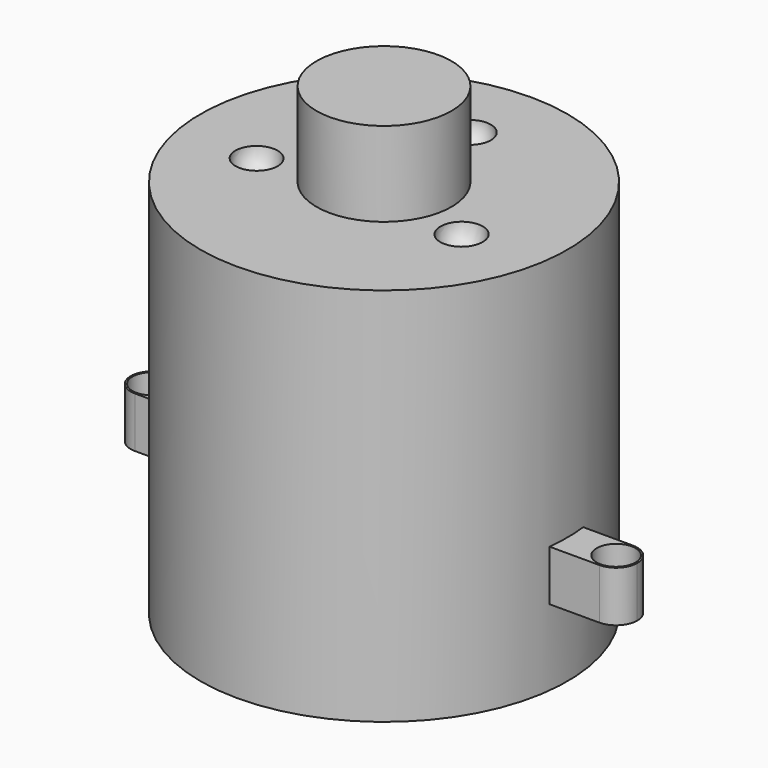
from build123d import *

# Parameters (mm, degrees)
F0_W     = 8
F0_H     = 10
F2_W     = 60
F2_H     = 6
F3_DEPTH = 2.5
F4_R     = 2.49999
F6_D     = 4.6
F6_DEPTH = 4
F6_TIP   = 1.3819794238


# Not quite as in the source:
# - a fillet or chamfer is up to 0.001 mm smaller than in the source, because OpenCascade refuses the exact size


with BuildPart() as f1:
    # F0 (on Right) → F1 (revolve)
    with BuildSketch(Plane.YZ):
        Polygon((-21.75, 22.5), (-21.75, -22.5), (0, -22.5), (0, 22.5), (-8, 22.5), align=None)
        with Locations((-4, 27.5)):
            Rectangle(F0_W, F0_H)
    revolve(axis=Axis((0, 0, 5), (0, 0, -1)))

    # F2 (on Front) → F3 (join, symmetric)
    with BuildSketch(Plane.XZ):
        with Locations((0, -10.5)):
            Rectangle(F2_W, F2_H)
    extrude(amount=F3_DEPTH, both=True)

    # F4 (radius 2.5 in the source; OpenCascade refuses exactly that, so slightly less here)
    f4_edges = [f1.edges().sort_by_distance(p)[0] for p in [
        (30, 2.5, -10.5),
        (-30, 2.5, -10.5),
        (30, -2.5, -10.5),
        (-30, -2.5, -10.5),
    ]]
    fillet(f4_edges, radius=F4_R)

    # F6
    with Locations(Plane.XY.offset(-7.5)):
        with Locations((-27.5, 0), (27.5, 0)):
            Hole(F6_D / 2, depth=F6_DEPTH)
            with Locations((0, 0, -(F6_DEPTH + F6_TIP / 2))):  # 118° drill point
                Cone(0, F6_D / 2, F6_TIP, mode=Mode.SUBTRACT)

    # F7 (on face) → F8 (revolve, cut)
    with BuildSketch(Plane.XY.offset(22.5)):
        with BuildLine():
            ThreePointArc((0, 10.197782052), (1.767766953, 10.9300150991), (2.5, 12.697782052))
            ThreePointArc((2.5, 12.697782052), (1.767766953, 14.465549005), (0, 15.197782052))
            Line((0, 15.197782052), (0, 10.197782052))
        make_face()
    revolve(axis=Axis((0, 12.697782052, 22.5), (0, -1, 0)), mode=Mode.SUBTRACT)

    # F7 (on face) → F9 (revolve, cut)
    with BuildSketch(Plane.XY.offset(22.5)):
        with BuildLine():
            Line((-14.6499237033, -3.669800331), (-9.65, -3.6893317878))
            ThreePointArc((-9.65, -3.6893317878), (-12.1402341971, -1.1893508621), (-14.6499237033, -3.669800331))
        make_face()
    revolve(axis=Axis((-12.1499618516, -3.6795660594, 22.5), (0.9999923703, -0.0039063212, 0)), mode=Mode.SUBTRACT)

    # F7 (on face) → F10 (revolve, cut)
    with BuildSketch(Plane.XY.offset(22.5)):
        with BuildLine():
            Line((9.6501744203, -3.7188626372), (14.65, -3.6893317878))
            ThreePointArc((14.65, -3.6893317878), (12.1352343178, -1.1893753933), (9.6501744203, -3.7188626372))
        make_face()
    revolve(axis=Axis((12.1500872101, -3.7040972125, 22.5), (0.9999825578, 0.0059062729, 0)), mode=Mode.SUBTRACT)


solid = f1.part
